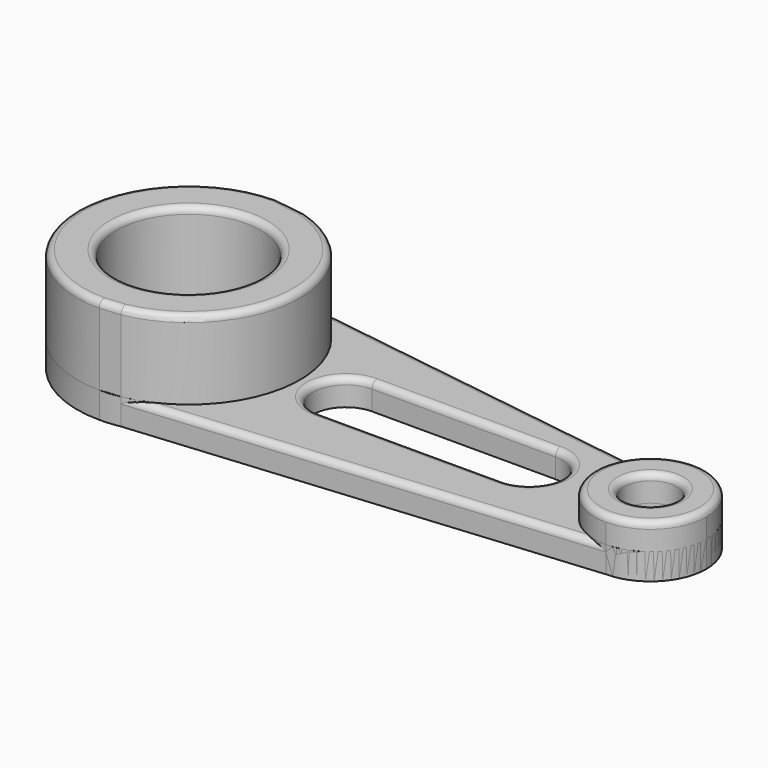
from build123d import *

# Parameters (mm, degrees)
F0_R           = 34.925
F1_DEPTH       = 50.8
F0_R_2         = 12.7
F2_DEPTH       = 25.4
F3_DEPTH       = 12.7
F4_T1_DEPTH    = 57.473964465
F4_T3_DEPTH    = 42.3670095889
F4_T6_ANGLE    = 196.8788005765
F4_T8_ANGLE    = 170.0203734018
F4_3_T1_DEPTH  = 88.9
F4_3_T6_DEPTH  = 267.3334584143
F4_3_S7_R      = 53.975
F4_3_T8_DEPTH  = 135
F4_3_S9_R      = 27.051
F4_3_T10_DEPTH = 135
F4_3_T12_ANGLE = 180
F4_3_T14_ANGLE = 180
F4_3_T18_DEPTH = 279.0764047625
F4_3_S19_R     = 27.051
F4_3_T20_DEPTH = 142
F4_3_S21_R     = 53.975
F4_3_T22_DEPTH = 142


# Not quite as in the source:
# - a fillet or chamfer that OpenCascade refuses, or shapes differently, is made with other operations: its cross-section is extruded or revolved along the edge and cut away or added


with BuildPart() as f1:
    # F0 (on Top) → F1 (new body)
    with BuildSketch(Plane.XY):
        with BuildLine():
            Line((-149.8773723314, 51.7838993497), (-165.1, 53.975))
            ThreePointArc((-165.1, 53.975), (-219.075, 0), (-165.1, -53.975))
            Line((-165.1, -53.975), (-155.292112943, -53.0764163869))
            ThreePointArc((-155.292112943, -53.0764163869), (-123.6109572965, -34.5247731426), (-111.125, 0))
            ThreePointArc((-111.125, 0), (-121.8857549331, 32.3392895453), (-149.8773723314, 51.7838993497))
        make_face()
        with Locations((-165.1, 0)):
            Circle(F0_R, mode=Mode.SUBTRACT)
    extrude(amount=F1_DEPTH)

    # F4: fillet of radius 3.175 on 5 edges, made by hand

    # F4_s2 → F4_t1 (cut)
    with BuildSketch(Plane(origin=(-192.3428235829, -17.6221553493, 0), x_dir=(0, 0, 1), z_dir=(0.9958292663, 0.0912363545, 0))):
        with BuildLine():
            ThreePointArc((50.8, 35.5117625257), (49.8700640303, 37.7568265559), (47.625, 38.6867625257))
            Line((47.625, 38.6867625257), (50.8, 38.6867625257))
            Line((50.8, 38.6867625257), (50.8, 35.5117625257))
        make_face()
    extrude(amount=F4_T1_DEPTH, mode=Mode.SUBTRACT)

    # F4_s4 → F4_t3 (cut)
    with BuildSketch(Plane(origin=(-140.7814868868, 20.2636768223, 0), x_dir=(0, 0, 1), z_dir=(-0.9897992898, 0.1424688244, 0))):
        with BuildLine():
            ThreePointArc((47.625, 29.9028137663), (49.8700640303, 28.9728777965), (50.8, 26.7278137663))
            Line((50.8, 26.7278137663), (50.8, 29.9028137663))
            Line((50.8, 29.9028137663), (47.625, 29.9028137663))
        make_face()
    extrude(amount=F4_T3_DEPTH, mode=Mode.SUBTRACT)

    # F4_s5 → F4_t6 (revolve, cut)
    with BuildSketch(Plane(origin=(-161.5438350134, 23.9682400245, 0), x_dir=(0, 0, 1), z_dir=(0.9891716429, -0.1467632817, 0))):
        with BuildLine():
            ThreePointArc((50.8, -26.5693821935), (49.8700640303, -28.8144462238), (47.625, -29.7443821935))
            Line((47.625, -29.7443821935), (50.8, -29.7443821935))
            Line((50.8, -29.7443821935), (50.8, -26.5693821935))
        make_face()
    revolve(axis=Axis((-165.1, 0, 50.8), (0, 0, 1)), revolution_arc=F4_T6_ANGLE, mode=Mode.SUBTRACT)

    # F4_s7 → F4_t8 (revolve, cut)
    with BuildSketch(Plane(origin=(-161.9450539773, 22.6037143836, 0), x_dir=(0, 0, 1), z_dir=(-0.9903992611, 0.1382364047, 0))):
        with BuildLine():
            ThreePointArc((50.8, 27.9771695808), (49.8700640303, 30.2222336111), (47.625, 31.1521695808))
            Line((47.625, 31.1521695808), (50.8, 31.1521695808))
            Line((50.8, 31.1521695808), (50.8, 27.9771695808))
        make_face()
    revolve(axis=Axis((-165.1, 0, 50.8), (0, 0, -1)), revolution_arc=F4_T8_ANGLE, mode=Mode.SUBTRACT)

    # F4_s9 → F4_t10 (revolve, cut)
    with BuildSketch(Plane.XZ):
        with BuildLine():
            ThreePointArc((-127, 50.8), (-129.2450640303, 49.8700640303), (-130.175, 47.625))
            Line((-130.175, 47.625), (-130.175, 50.8))
            Line((-130.175, 50.8), (-127, 50.8))
        make_face()
    revolve(axis=Axis((-165.1, 0, 50.8), (0, 0, 1)), mode=Mode.SUBTRACT)


with BuildPart() as f2:
    # F0 (on Top) → F2 (new body)
    with BuildSketch(Plane.XY):
        with BuildLine():
            ThreePointArc((90.551, -5.980017595), (82.6279455379, 13.1479279429), (63.5, 21.070982405))
            ThreePointArc((63.5, 21.070982405), (36.449, -5.980017595), (63.5, -33.031017595))
            ThreePointArc((63.5, -33.031017595), (82.6279455379, -25.1079631329), (90.551, -5.980017595))
        make_face()
        with Locations((63.5, -5.980017595)):
            Circle(F0_R_2, mode=Mode.SUBTRACT)
    extrude(amount=F2_DEPTH)

    # F4#2: fillet of radius 3.175 on 2 edges, made by hand

    # F4_2_s1 → F4_2_t2 (revolve, cut)
    with BuildSketch(Plane.YZ.offset(63.5)):
        with BuildLine():
            ThreePointArc((-33.031017595, 22.225), (-32.1010816253, 24.4700640303), (-29.856017595, 25.4))
            Line((-29.856017595, 25.4), (-33.031017595, 25.4))
            Line((-33.031017595, 25.4), (-33.031017595, 22.225))
        make_face()
    revolve(axis=Axis((63.5, -5.980017595, 25.4), (0, 0, -1)), mode=Mode.SUBTRACT)

    # F4_2_s3 → F4_2_t4 (revolve, cut)
    with BuildSketch(Plane.XZ.offset(5.980017595)):
        with BuildLine():
            ThreePointArc((79.375, 25.4), (77.1299359697, 24.4700640303), (76.2, 22.225))
            Line((76.2, 22.225), (76.2, 25.4))
            Line((76.2, 25.4), (79.375, 25.4))
        make_face()
    revolve(axis=Axis((63.5, -5.980017595, 25.4), (0, 0, 1)), mode=Mode.SUBTRACT)


with BuildPart() as f3:
    # F0 (on Top) → F3 (new body)
    with BuildSketch(Plane.XY):
        with BuildLine():
            Line((-149.8773723314, 51.7838993497), (-165.1, 53.975))
            ThreePointArc((-165.1, 53.975), (-219.075, 0), (-165.1, -53.975))
            Line((-165.1, -53.975), (-155.292112943, -53.0764163869))
            ThreePointArc((-155.292112943, -53.0764163869), (-123.6109572965, -34.5247731426), (-111.125, 0))
            ThreePointArc((-111.125, 0), (-121.8857549331, 32.3392895453), (-149.8773723314, 51.7838993497))
        make_face()
        with Locations((-165.1, 0)):
            Circle(F0_R, mode=Mode.SUBTRACT)
        with BuildLine():
            ThreePointArc((-149.8773723314, 51.7838993497), (-157.4102452056, 53.4244166669), (-165.1, 53.975))
            Line((-165.1, 53.975), (-149.8773723314, 51.7838993497))
        make_face()
        with BuildLine():
            Line((-155.3437359105, -53.0859297368), (-165.1, -53.975))
            ThreePointArc((-165.1, -53.975), (-160.201655001, -53.752272894), (-155.3437359105, -53.0859297368))
        make_face()
        with BuildLine():
            Line((-155.292112943, -53.0764163869), (-165.1, -53.975))
            Line((-165.1, -53.975), (-155.3437359105, -53.0859297368))
            ThreePointArc((-155.3437359105, -53.0859297368), (-155.3179232702, -53.0811793374), (-155.292112943, -53.0764163869))
        make_face()
        with BuildLine():
            Line((63.5, 21.070982405), (-149.8773723314, 51.7838993497))
            ThreePointArc((-149.8773723314, 51.7838993497), (-121.8857549331, 32.3392895453), (-111.125, 0))
            ThreePointArc((-111.125, 0), (-123.6109572965, -34.5247731426), (-155.292112943, -53.0764163869))
            Line((-155.292112943, -53.0764163869), (63.5, -33.031017595))
            ThreePointArc((63.5, -33.031017595), (36.449, -5.980017595), (63.5, 21.070982405))
        make_face()
        with BuildLine():
            ThreePointArc((0, 15.875), (15.875, 0), (0, -15.875))
            Line((0, -15.875), (-88.9, -15.875))
            ThreePointArc((-88.9, -15.875), (-104.775, 0), (-88.9, 15.875))
            Line((-88.9, 15.875), (0, 15.875))
        make_face(mode=Mode.SUBTRACT)
        with BuildLine():
            ThreePointArc((90.551, -5.980017595), (82.6279455379, 13.1479279429), (63.5, 21.070982405))
            ThreePointArc((63.5, 21.070982405), (36.449, -5.980017595), (63.5, -33.031017595))
            ThreePointArc((63.5, -33.031017595), (82.6279455379, -25.1079631329), (90.551, -5.980017595))
        make_face()
        with Locations((63.5, -5.980017595)):
            Circle(F0_R_2, mode=Mode.SUBTRACT)
    extrude(amount=F3_DEPTH)

    # F4#3: fillet of radius 3.175 on 6 edges, made by hand

    # F4_3_s2 → F4_3_t1 (cut)
    with BuildSketch(Plane.YZ.offset(-88.9)):
        with BuildLine():
            ThreePointArc((-15.875, 9.525), (-16.8049359697, 11.7700640303), (-19.05, 12.7))
            Line((-19.05, 12.7), (-15.875, 12.7))
            Line((-15.875, 12.7), (-15.875, 9.525))
        make_face()
        with BuildLine():
            ThreePointArc((15.875, 9.525), (16.8049359697, 11.7700640303), (19.05, 12.7))
            Line((19.05, 12.7), (15.875, 12.7))
            Line((15.875, 12.7), (15.875, 9.525))
        make_face()
    extrude(amount=F4_3_T1_DEPTH, mode=Mode.SUBTRACT)


with BuildPart() as f4_3_tool4:
    # F4_3_s5 → F4_3_t6 (new body)
    with BuildSketch(Plane(origin=(-182.5349365259, -16.7235717362, 0), x_dir=(0, 0, 1), z_dir=(0.9958292663, 0.0912363545, 0))):
        with BuildLine():
            ThreePointArc((9.525, 38.6867625257), (11.7700640303, 37.7568265559), (12.7, 35.5117625257))
            Line((12.7, 35.5117625257), (12.7, 38.6867625257))
            Line((12.7, 38.6867625257), (9.525, 38.6867625257))
        make_face()
    extrude(amount=F4_3_T6_DEPTH)

    # F4_3_s7 → F4_3_t8 (cut, symmetric)
    with BuildSketch(Plane.XY.offset(11.1)):
        with Locations((-165.1, 0)):
            Circle(F4_3_S7_R)
    extrude(amount=F4_3_T8_DEPTH, both=True, mode=Mode.SUBTRACT)

    # F4_3_s9 → F4_3_t10 (cut, symmetric)
    with BuildSketch(Plane.XY.offset(11.1)):
        with Locations((63.5, -5.980017595)):
            Circle(F4_3_S9_R)
    extrude(amount=F4_3_T10_DEPTH, both=True, mode=Mode.SUBTRACT)


with BuildPart() as f3_1:
    add(f3.part)

    # F4_3_t3: cut F4_3_tool4
    add(f4_3_tool4.part, mode=Mode.SUBTRACT)

    # F4_3_s11 → F4_3_t12 (revolve, cut)
    with BuildSketch(Plane.YZ.offset(-88.9)):
        with BuildLine():
            ThreePointArc((-15.875, 9.525), (-16.8049359697, 11.7700640303), (-19.05, 12.7))
            Line((-19.05, 12.7), (-15.875, 12.7))
            Line((-15.875, 12.7), (-15.875, 9.525))
        make_face()
    revolve(axis=Axis((-88.9, 0, 12.7), (0, 0, -1)), revolution_arc=F4_3_T12_ANGLE, mode=Mode.SUBTRACT)

    # F4_3_s13 → F4_3_t14 (revolve, cut)
    with BuildSketch(Plane.YZ):
        with BuildLine():
            ThreePointArc((15.875, 9.525), (16.8049359697, 11.7700640303), (19.05, 12.7))
            Line((19.05, 12.7), (15.875, 12.7))
            Line((15.875, 12.7), (15.875, 9.525))
        make_face()
    revolve(axis=Axis((0, 0, 12.7), (0, 0, -1)), revolution_arc=F4_3_T14_ANGLE, mode=Mode.SUBTRACT)


with BuildPart() as f4_3_tool16:
    # F4_3_s17 → F4_3_t18 (new body)
    with BuildSketch(Plane(origin=(82.8093768662, -11.9193403037, 0), x_dir=(0, 0, 1), z_dir=(-0.9897992898, 0.1424688244, 0))):
        with BuildLine():
            ThreePointArc((9.525, 29.9028137663), (11.7700640303, 28.9728777965), (12.7, 26.7278137663))
            Line((12.7, 26.7278137663), (12.7, 29.9028137663))
            Line((12.7, 29.9028137663), (9.525, 29.9028137663))
        make_face()
    extrude(amount=F4_3_T18_DEPTH)

    # F4_3_s19 → F4_3_t20 (cut, symmetric)
    with BuildSketch(Plane.XY.offset(11.1)):
        with Locations((63.5, -5.980017595)):
            Circle(F4_3_S19_R)
    extrude(amount=F4_3_T20_DEPTH, both=True, mode=Mode.SUBTRACT)

    # F4_3_s21 → F4_3_t22 (cut, symmetric)
    with BuildSketch(Plane.XY.offset(11.1)):
        with Locations((-165.1, 0)):
            Circle(F4_3_S21_R)
    extrude(amount=F4_3_T22_DEPTH, both=True, mode=Mode.SUBTRACT)


with BuildPart() as f3_2:
    add(f3_1.part)

    # F4_3_t15: cut F4_3_tool16
    add(f4_3_tool16.part, mode=Mode.SUBTRACT)


solid = Compound([f1.part, f2.part, f3_2.part])
